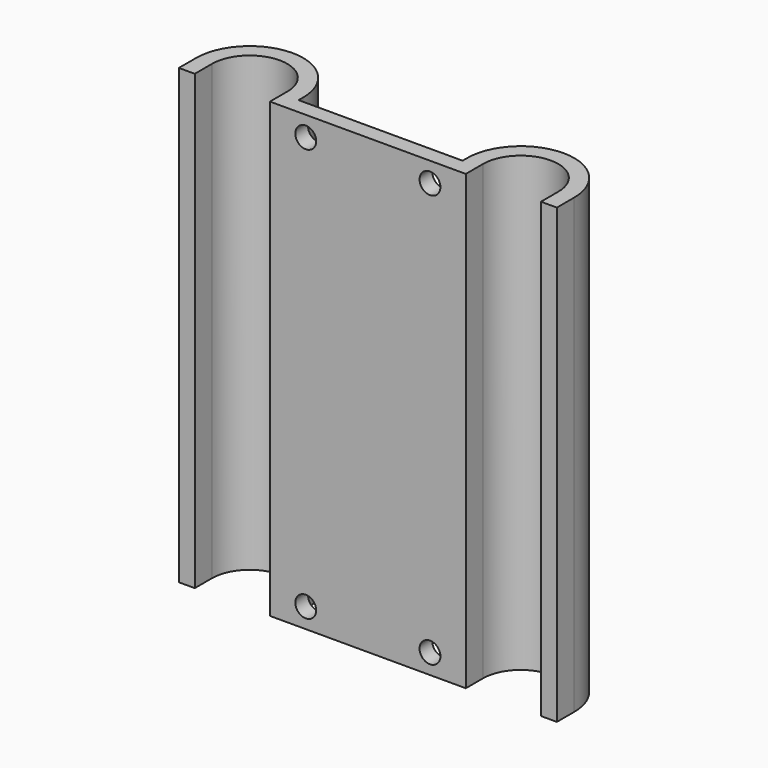
from build123d import *

# Parameters (mm, degrees)
F1_DEPTH = 90.3440154
F2_R     = 2.0828
F3_DEPTH = 3.175
F5_DEPTH = 20.240498
F6_SIZE  = 20.240488
F7_R     = 1.7272
F8_DEPTH = 4.7625


# Not quite as in the source:
# - a fillet or chamfer is up to 0.001 mm smaller than in the source, because OpenCascade refuses the exact size


with BuildPart() as f1:
    # F0 (on Top) → F1 (new body)
    with BuildSketch(Plane.XY):
        with BuildLine():
            Line((32.7249998, 0), (0, 0))
            Line((0, 0), (0, 1.1500104))
            ThreePointArc((0, 1.1500104), (-10.675, 11.8250104), (-21.35, 1.1500104))
            Line((-21.35, 1.1500104), (-21.35, -3.175))
            Line((-21.35, -3.175), (-18.175, -3.175))
            Line((-18.175, -3.175), (-18.175, 1.1500104))
            ThreePointArc((-18.175, 1.1500104), (-10.675, 8.6500104), (-3.175, 1.1500104))
            Line((-3.175, 1.1500104), (-3.175, -3.175))
            Line((-3.175, -3.175), (35.8999998, -3.175))
            Line((35.8999998, -3.175), (35.8999998, 1.1500104))
            ThreePointArc((35.8999998, 1.1500104), (43.3999998, 8.6500104), (50.8999998, 1.1500104))
            Line((50.8999998, 1.1500104), (50.8999998, -3.175))
            Line((50.8999998, -3.175), (54.0749998, -3.175))
            Line((54.0749998, -3.175), (54.0749998, 1.1500104))
            ThreePointArc((54.0749998, 1.1500104), (43.3999998, 11.8250104), (32.7249998, 1.1500104))
            Line((32.7249998, 1.1500104), (32.7249998, 0))
        make_face()
    extrude(amount=F1_DEPTH)

    # F2 (on face) → F3 (cut, through all)
    with BuildSketch(Plane(origin=(0, 0, 0), x_dir=(-1, 0, 0), z_dir=(0, 1, 0))):
        with Locations((-3.96875, 3.96875)):
            Circle(F2_R)
        with Locations((-28.7562498, 3.96875)):
            Circle(F2_R)
        with Locations((-28.7562498, 86.3752654)):
            Circle(F2_R)
        with Locations((-3.96875, 86.3752654)):
            Circle(F2_R)
    extrude(amount=-F3_DEPTH, mode=Mode.SUBTRACT)

    # F4 (on face) → F5 (join)
    with BuildSketch(Plane(origin=(0, 0, 0), x_dir=(-1, 0, 0), z_dir=(0, 1, 0))):
        Polygon((-25.8874999, 55.52801188), (-25.8874999, 30.52501388), (-6.8374999, 30.52501388), (-6.8374999, 55.52801188), (-11.5999999, 55.52801188), (-11.5999999, 35.28751388), (-21.1249999, 35.28751388), (-21.1249999, 55.52801188), align=None)
    extrude(amount=F5_DEPTH)

    # F6 (size 20.240498 in the source; OpenCascade refuses exactly that, so slightly less here)
    f6_edges = [f1.edges().sort_by_distance(p)[0] for p in [
        (23.50625, 20.240498, 55.528012),
        (9.21875, 20.240498, 55.528012),
    ]]
    chamfer(f6_edges, length=F6_SIZE)

    # F7 (on face) → F8 (cut, through all)
    with BuildSketch(Plane.XY.offset(35.28751388)):
        with Locations((16.3624999, 15.477998)):
            Circle(F7_R)
    extrude(amount=-F8_DEPTH, mode=Mode.SUBTRACT)


solid = f1.part
